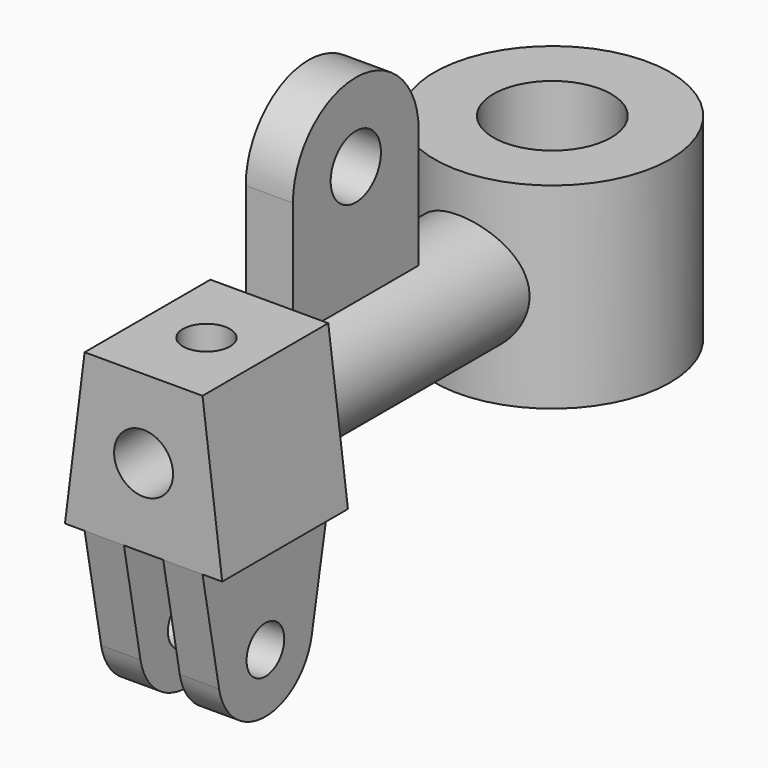
from build123d import *

# Parameters (mm, degrees)
F1_DEPTH  = 40
F2_R      = 15
F3_DEPTH  = 90
F4_R      = 30
F5_DEPTH  = 25
F6_R      = 8
F7_DEPTH  = 6
F10_DEPTH = 10
F11_R     = 6
F12_DEPTH = 10
F13_R     = 15
F14_DEPTH = 85.001
F15_R     = 6
F16_DEPTH = 8
F17_R     = 7.5
F18_DEPTH = 110


# Not quite as in the source:
# - a pattern or mirror of a feature is missing from the dataset's text; its kind, count and spacing are read off the source's solid


with BuildPart() as f1:
    # F0 (on Front) → F1 (new body)
    with BuildSketch(Plane.XZ):
        Polygon((15, 20), (-15, 20), (-20, -20), (20, -20), align=None)
    extrude(amount=-F1_DEPTH)

    # F2 (on face) → F3 (join)
    with BuildSketch(Plane(origin=(0, 40, 0), x_dir=(-1, 0, 0), z_dir=(0, 1, 0))):
        Circle(F2_R)
    extrude(amount=F3_DEPTH)

    # F4 (on Top) → F5 (join, symmetric)
    with BuildSketch(Plane.XY):
        with Locations((0, 130)):
            Circle(F4_R)
    extrude(amount=F5_DEPTH, both=True)

    # F6 (on Right) → F7 (join, symmetric)
    with BuildSketch(Plane.YZ):
        with BuildLine():
            Line((40, 44), (40, 10.4397451505))
            Line((40, 10.4397451505), (40, 6.8427645601))
            Line((40, 6.8427645601), (80, 6.8427645601))
            Line((80, 6.8427645601), (80, 44))
            ThreePointArc((80, 44), (60, 64), (40, 44))
        make_face()
        with Locations((60, 44)):
            Circle(F6_R, mode=Mode.SUBTRACT)
    extrude(amount=F7_DEPTH, both=True)

    # F9 (on offset) → F10 (join)
    with BuildSketch(Plane.YZ.offset(15)):
        with BuildLine():
            Line((0, -20), (5.2618519826, -47.7905184139))
            ThreePointArc((5.2618519826, -47.7905184139), (20, -60), (34.7381480174, -47.7905184139))
            Line((34.7381480174, -47.7905184139), (40, -20))
            Line((40, -20), (0, -20))
        make_face()
    f10 = extrude(amount=-F10_DEPTH)

    # F10_copies: F10 across plane
    add(f10.mirror(Plane(origin=(0, 0, 0), x_dir=(0, 0, -1), z_dir=(-1, 0, 0))))

    # F11 (on face) → F12 (cut, through all)
    with BuildSketch(Plane.YZ.offset(15)):
        with Locations((20, -45)):
            Circle(F11_R)
    f12 = extrude(amount=-F12_DEPTH, mode=Mode.SUBTRACT)

    # F12_copies: F12 across plane
    add(f12.mirror(Plane(origin=(0, 0, 0), x_dir=(0, 0, -1), z_dir=(-1, 0, 0))), mode=Mode.SUBTRACT)

    # F13 (on face) → F14 (cut, through all)
    with BuildSketch(Plane.XY.offset(25)):
        with Locations((0, 130)):
            Circle(F13_R)
    extrude(amount=-F14_DEPTH, mode=Mode.SUBTRACT)

    # F15 (on face) → F16 (cut)
    with BuildSketch(Plane.XY.offset(20)):
        with Locations((0, 20)):
            Circle(F15_R)
    extrude(amount=-F16_DEPTH, mode=Mode.SUBTRACT)

    # F17 (on face) → F18 (cut)
    with BuildSketch(Plane.XZ):
        Circle(F17_R)
    extrude(amount=-F18_DEPTH, mode=Mode.SUBTRACT)


solid = f1.part
